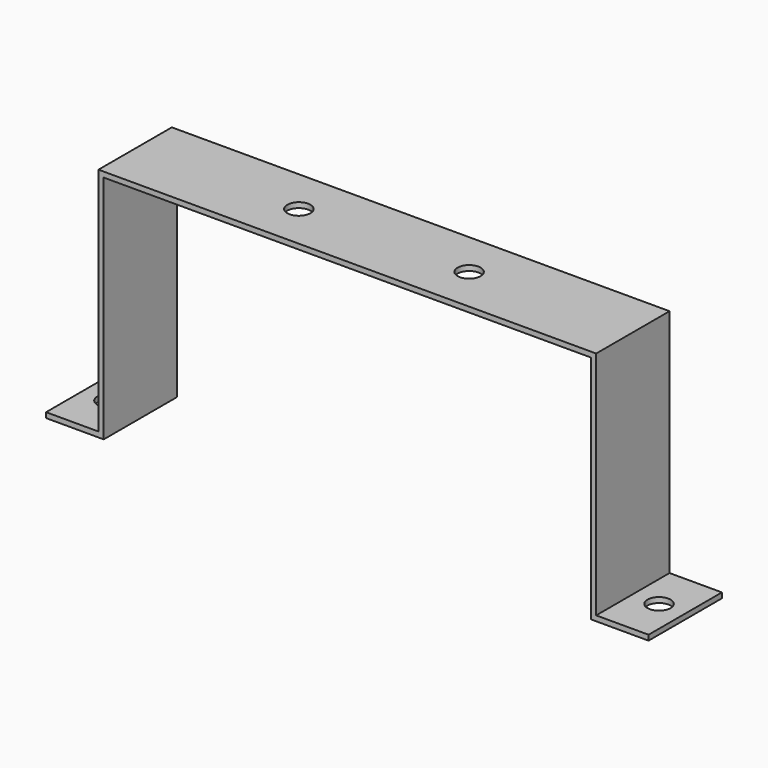
from build123d import *

# Parameters (mm, degrees)
F1_DEPTH = 17.5
F2_R     = 4.4
F3_DEPTH = 25
F4_R     = 4.4
F5_DEPTH = 25


# Not quite as in the source:
# - a feature names something its author has since deleted; it is built from what else it names


with BuildPart() as f1:
    # F0 (on Front) → F1 (new body, symmetric)
    with BuildSketch(Plane.XZ):
        Polygon((95, -38), (95, 50), (-95, 50), (-95, -38), (-115, -38), (-115, -40), (-93, -40), (-93, 48), (93, 48), (93, -40), (115, -40), (115, -38), align=None)
    extrude(amount=F1_DEPTH, both=True)

    # F2 (on face) → F3 (cut)
    with BuildSketch(Plane.XY.offset(-38)):
        with Locations((-105, 0)):
            Circle(F2_R)
        with Locations((105, 0)):
            Circle(F2_R)
    extrude(amount=-F3_DEPTH, mode=Mode.SUBTRACT)

    # F4 (on face) → F5 (cut)
    with BuildSketch(Plane.XY.offset(50)):
        with Locations((-32.5, 0)):
            Circle(F4_R)
        with Locations((32.5, 0)):
            Circle(F4_R)
    extrude(amount=-F5_DEPTH, mode=Mode.SUBTRACT)


solid = f1.part
